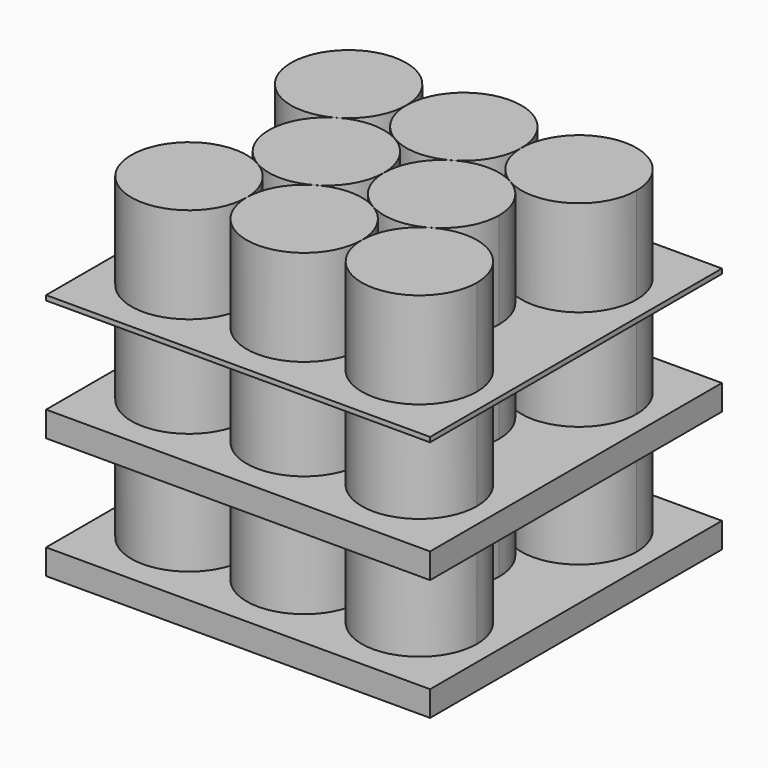
from build123d import *

# Parameters (mm, degrees)
F1_DEPTH = 84.1627984
F2_W     = 101.6
F2_H     = 6.6927933697
F3_DEPTH = 48.26
F2_H_2   = 6.6927984
F2_H_3   = 1.27


# Not quite as in the source:
# - a feature names something its author has since deleted; it is built from what else it names


with BuildPart() as f1:
    # F0 (on Top) → F1 (new body)
    with BuildSketch(Plane.XY):
        with BuildLine():
            ThreePointArc((-22.8599997596, -13.1982272925), (-43.6782272231, -34.0164541872), (-15.24, -26.3964543073))
            ThreePointArc((-15.24, -26.3964543073), (-17.2817727769, -18.7764544275), (-22.8599997596, -13.1982272925))
        make_face()
    extrude(amount=F1_DEPTH)


with BuildPart() as f1b:
    # F0 (on Top) → F1, piece 2 (new body)
    with BuildSketch(Plane.XY):
        with BuildLine():
            ThreePointArc((-7.6199998958, -13.1982270935), (-13.1982271236, -18.7764542553), (-15.24, -26.3964543073))
            ThreePointArc((-15.24, -26.3964543073), (0, -41.6364543073), (15.24, -26.3964543073))
            ThreePointArc((15.24, -26.3964543073), (13.1982272501, -18.7764544743), (7.6200003339, -13.1982273465))
            ThreePointArc((7.6200003339, -13.1982273465), (2.529e-07, -11.1564543073), (-7.6199998958, -13.1982270935))
        make_face()
    extrude(amount=F1_DEPTH)


with BuildPart() as f1c:
    # F0 (on Top) → F1, piece 3 (new body)
    with BuildSketch(Plane.XY):
        with BuildLine():
            ThreePointArc((-22.8600001039, 13.1982270937), (-30.48, -1.988e-07), (-22.8599997596, -13.1982272925))
            ThreePointArc((-22.8599997596, -13.1982272925), (-15.2399998011, -15.24), (-7.6199998958, -13.1982270935))
            ThreePointArc((-7.6199998958, -13.1982270935), (-2.0417728163, -7.6199999479), (0, 0))
            ThreePointArc((0, 0), (-2.0417727499, 7.619999833), (-7.6199996661, 13.1982269609))
            ThreePointArc((-7.6199996661, 13.1982269609), (-15.2399998672, 15.24), (-22.8600001039, 13.1982270937))
        make_face()
    extrude(amount=F1_DEPTH)


with BuildPart() as f1d:
    # F0 (on Top) → F1, piece 4 (new body)
    with BuildSketch(Plane.XY):
        with BuildLine():
            ThreePointArc((22.8599997751, -13.1982272835), (17.2817727814, -18.7764544198), (15.24, -26.3964543073))
            ThreePointArc((15.24, -26.3964543073), (30.48, -41.6364543073), (45.72, -26.3964543073))
            ThreePointArc((45.72, -26.3964543073), (38.0999998875, -13.1982270887), (22.8599997751, -13.1982272835))
        make_face()
    extrude(amount=F1_DEPTH)


with BuildPart() as f1e:
    # F0 (on Top) → F1, piece 5 (new body)
    with BuildSketch(Plane.XY):
        with BuildLine():
            ThreePointArc((-15.24, 26.3964543073), (-43.6782271237, 34.0164543593), (-22.8600001039, 13.1982270937))
            ThreePointArc((-22.8600001039, 13.1982270937), (-17.2817728763, 18.7764542554), (-15.24, 26.3964543073))
        make_face()
    extrude(amount=F1_DEPTH)


with BuildPart() as f1f:
    # F0 (on Top) → F1, piece 6 (new body)
    with BuildSketch(Plane.XY):
        with BuildLine():
            ThreePointArc((0, 0), (2.0417729427, -7.620000167), (7.6200003339, -13.1982273465))
            ThreePointArc((7.6200003339, -13.1982273465), (15.2400000629, -15.24), (22.8599997751, -13.1982272835))
            ThreePointArc((22.8599997751, -13.1982272835), (28.4382270887, -7.6200001125), (30.48, 0))
            ThreePointArc((30.48, 0), (28.4382272477, 7.6199998371), (22.8600003259, 13.1982269655))
            ThreePointArc((22.8600003259, 13.1982269655), (15.2400002483, 15.24), (7.6200001042, 13.1982272138))
            ThreePointArc((7.6200001042, 13.1982272138), (2.0417728764, 7.6200000521), (0, 0))
        make_face()
    extrude(amount=F1_DEPTH)


with BuildPart() as f1g:
    # F0 (on Top) → F1, piece 7 (new body)
    with BuildSketch(Plane.XY):
        with BuildLine():
            ThreePointArc((-15.24, 26.3964543073), (-13.1982270573, 18.7764541404), (-7.6199996661, 13.1982269609))
            ThreePointArc((-7.6199996661, 13.1982269609), (2.529e-07, 11.1564543073), (7.6200001042, 13.1982272138))
            ThreePointArc((7.6200001042, 13.1982272138), (13.1982271837, 18.7764543594), (15.24, 26.3964543073))
            ThreePointArc((15.24, 26.3964543073), (0, 41.6364543073), (-15.24, 26.3964543073))
        make_face()
    extrude(amount=F1_DEPTH)


with BuildPart() as f1h:
    # F0 (on Top) → F1, piece 8 (new body)
    with BuildSketch(Plane.XY):
        with BuildLine():
            ThreePointArc((45.72, 26.3964543073), (30.48, 41.6364543073), (15.24, 26.3964543073))
            ThreePointArc((15.24, 26.3964543073), (17.2817729404, 18.7764541444), (22.8600003259, 13.1982269655))
            ThreePointArc((22.8600003259, 13.1982269655), (38.1000001629, 13.1982272477), (45.72, 26.3964543073))
        make_face()
    extrude(amount=F1_DEPTH)


with BuildPart() as f3:
    # F2 (on Front) → F3 (new body, symmetric)
    with BuildSketch(Plane.XZ):
        with Locations((0, -3.3463966849)):
            Rectangle(F2_W, F2_H)
    extrude(amount=F3_DEPTH, both=True)


with BuildPart() as f3b:
    # F2 (on Front) → F3, piece 2 (new body, symmetric)
    with BuildSketch(Plane.XZ):
        with Locations((0, 28.7463992)):
            Rectangle(F2_W, F2_H_2)
    extrude(amount=F3_DEPTH, both=True)


with BuildPart() as f3c:
    # F2 (on Front) → F3, piece 3 (new body, symmetric)
    with BuildSketch(Plane.XZ):
        with Locations((0, 58.1277984)):
            Rectangle(F2_W, F2_H_3)
    extrude(amount=F3_DEPTH, both=True)


solid = Compound([f1.part, f1b.part, f1c.part, f1d.part, f1e.part, f1f.part, f1g.part, f1h.part, f3.part, f3b.part, f3c.part])
